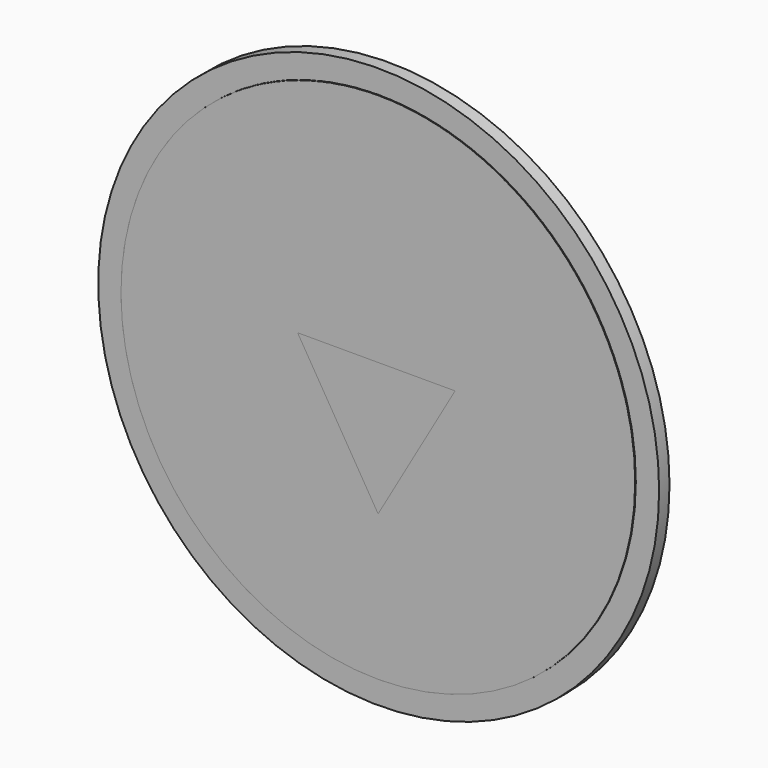
from build123d import *

# Parameters (mm, degrees)
F3_DEPTH  = 2.54
F1_R      = 52.0612504087
F4_DEPTH  = 2.4054199457
F3_FACE_R = 47.7269460656
F5_DEPTH  = 0.5445368588
F5_TAPER  = -3


with BuildPart() as f3:
    # F0 (on Front) → F3 (new body)
    with BuildSketch(Plane.XZ):
        Polygon((14.2906159163, 4.056841135), (43.6209606961, 19.3668058466), (-43.6209606961, 19.3668058466), (-14.9385407567, 4.056841135), align=None)
        with BuildLine():
            ThreePointArc((0, -47.7269460656), (33.7480472083, -33.7480472083), (47.7269460656, 0))
            ThreePointArc((47.7269460656, 0), (46.6891669406, 9.8986398631), (43.6209606961, 19.3668058466))
            Line((43.6209606961, 19.3668058466), (0, -47.7269460656))
        make_face()
        with BuildLine():
            Line((-43.6209606961, 19.3668058466), (43.6209606961, 19.3668058466))
            ThreePointArc((43.6209606961, 19.3668058466), (0, 47.7269460656), (-43.6209606961, 19.3668058466))
        make_face()
        Polygon((0, -47.7269460656), (43.6209606961, 19.3668058466), (14.2906159163, 4.056841135), (0, -20.6848606467), align=None)
        with BuildLine():
            ThreePointArc((-43.6209606961, 19.3668058466), (-40.0136219234, -26.01483118), (0, -47.7269460656))
            Line((0, -47.7269460656), (-43.6209606961, 19.3668058466))
        make_face()
        Polygon((-43.6209606961, 19.3668058466), (0, -47.7269460656), (0, -20.6848606467), (-14.9385407567, 4.056841135), align=None)
    extrude(amount=F3_DEPTH)


with BuildPart() as f3b:
    # F2 (on Front) → F3, piece 2 (new body)
    with BuildSketch(Plane.XZ):
        Polygon((-32.3546789587, 14.0674561262), (0, -39.0817448497), (32.9583846033, 14.0674561262), align=None)
    extrude(amount=F3_DEPTH)


with BuildPart() as f4:
    # F1 (on Front) → F4 (new body)
    with BuildSketch(Plane.XZ):
        Circle(F1_R)
    extrude(amount=F4_DEPTH)


with BuildPart() as f4b:
    # F0 (on Front) → F4, piece 2 (new body)
    with BuildSketch(Plane.XZ):
        with BuildLine():
            ThreePointArc((0, -47.7269460656), (33.7480472083, -33.7480472083), (47.7269460656, 0))
            ThreePointArc((47.7269460656, 0), (46.6891669406, 9.8986398631), (43.6209606961, 19.3668058466))
            Line((43.6209606961, 19.3668058466), (0, -47.7269460656))
        make_face()
        with BuildLine():
            Line((-43.6209606961, 19.3668058466), (43.6209606961, 19.3668058466))
            ThreePointArc((43.6209606961, 19.3668058466), (0, 47.7269460656), (-43.6209606961, 19.3668058466))
        make_face()
        Polygon((14.2906159163, 4.056841135), (43.6209606961, 19.3668058466), (-43.6209606961, 19.3668058466), (-14.9385407567, 4.056841135), align=None)
        Polygon((0, -47.7269460656), (43.6209606961, 19.3668058466), (14.2906159163, 4.056841135), (0, -20.6848606467), align=None)
        with BuildLine():
            ThreePointArc((-43.6209606961, 19.3668058466), (-40.0136219234, -26.01483118), (0, -47.7269460656))
            Line((0, -47.7269460656), (-43.6209606961, 19.3668058466))
        make_face()
        Polygon((-43.6209606961, 19.3668058466), (0, -47.7269460656), (0, -20.6848606467), (-14.9385407567, 4.056841135), align=None)
    extrude(amount=F4_DEPTH)


with BuildPart() as f5:
    # F0 (on Front) + F3_face (on face) → F5 (new body)
    with BuildSketch(Plane.XZ):
        with BuildLine():
            ThreePointArc((0, -47.7269460656), (33.7480472083, -33.7480472083), (47.7269460656, 0))
            ThreePointArc((47.7269460656, 0), (46.6891669406, 9.8986398631), (43.6209606961, 19.3668058466))
            Line((43.6209606961, 19.3668058466), (0, -47.7269460656))
        make_face()
        with BuildLine():
            Line((-43.6209606961, 19.3668058466), (43.6209606961, 19.3668058466))
            ThreePointArc((43.6209606961, 19.3668058466), (0, 47.7269460656), (-43.6209606961, 19.3668058466))
        make_face()
        Polygon((14.2906159163, 4.056841135), (43.6209606961, 19.3668058466), (-43.6209606961, 19.3668058466), (-14.9385407567, 4.056841135), align=None)
        Polygon((0, -47.7269460656), (43.6209606961, 19.3668058466), (14.2906159163, 4.056841135), (0, -20.6848606467), align=None)
        with BuildLine():
            ThreePointArc((-43.6209606961, 19.3668058466), (-40.0136219234, -26.01483118), (0, -47.7269460656))
            Line((0, -47.7269460656), (-43.6209606961, 19.3668058466))
        make_face()
        Polygon((-43.6209606961, 19.3668058466), (0, -47.7269460656), (0, -20.6848606467), (-14.9385407567, 4.056841135), align=None)
    with BuildSketch(Plane(origin=(0.0114937106, -2.54, 0.2230034674), x_dir=(1, 0, 0), z_dir=(0, -1, 0))):
        with Locations((-0.0114937106, -0.2230034674)):
            Circle(F3_FACE_R)
        Polygon((-14.9500344673, 3.8338376676), (14.2791222057, 3.8338376676), (-0.0114937106, -20.9078641141), align=None, mode=Mode.SUBTRACT)
    extrude(amount=-F5_DEPTH, taper=F5_TAPER)


solid = Compound([f3.part, f3b.part, f4.part, f4b.part, f5.part])
